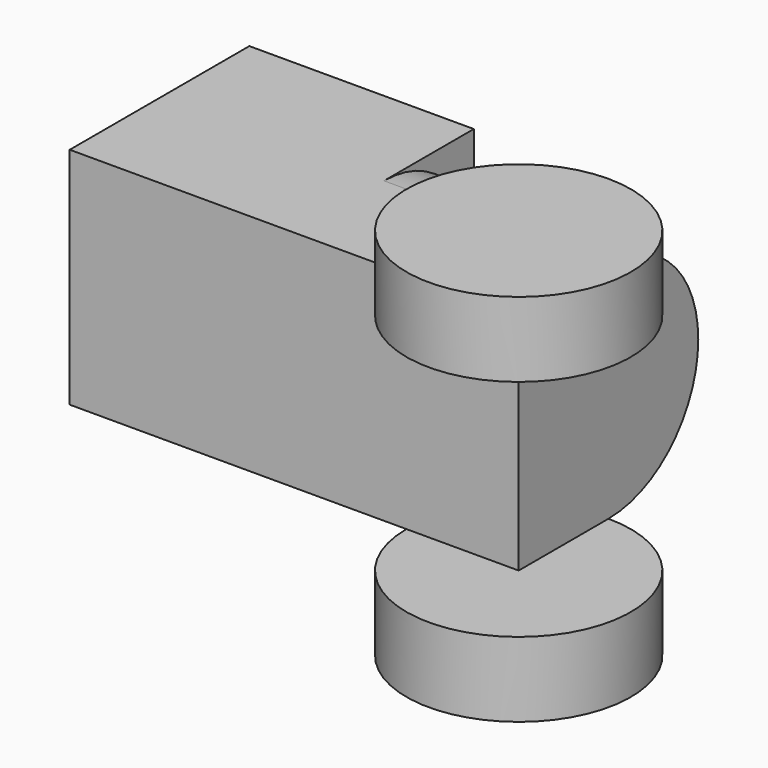
from build123d import *

# Parameters (mm, degrees)
F0_W     = 38.1
F0_H     = 38.1
F1_DEPTH = 38.1
F3_DEPTH = 38.1
F4_DEPTH = 19.05
F7_DEPTH = 12.7
F8_DEPTH = 12.7


# Not quite as in the source:
# - a feature of the source that left no trace in its solid (it failed there, or was rolled back) is left out


with BuildPart() as f1:
    # F0 (on Front) → F1 (new body)
    with BuildSketch(Plane.XZ):
        with Locations((-45.594806087, -5.8171211302)):
            Rectangle(F0_W, F0_H)
    extrude(amount=F1_DEPTH)

    # F2 (on face) → F3 (join)
    with BuildSketch(Plane.YZ.offset(-26.544806087)):
        with BuildLine():
            Line((-19.05, 13.2328788698), (-19.05, -24.8671211302))
            ThreePointArc((-19.05, -24.8671211302), (-5.5796158184, -19.2875053118), (0, -5.8171211302))
            ThreePointArc((0, -5.8171211302), (-5.5796158184, 7.6532630514), (-19.05, 13.2328788698))
        make_face()
    extrude(amount=F3_DEPTH)

    # F4 (add): a face of the model
    f4_faces = [f1.faces().sort_by_distance(p)[0] for p in [
        (-7.494806087, -19.05, -5.8171211302),
    ]]
    extrude(f4_faces, amount=F4_DEPTH)

    # F6 (on face) → F7 (join)
    with BuildSketch(Plane.XY.offset(13.2328788698)):
        with BuildLine():
            ThreePointArc((-7.494806087, -38.1), (11.555193913, -57.15), (30.605193913, -38.1))
            ThreePointArc((30.605193913, -38.1), (25.0255780946, -24.6296158184), (11.555193913, -19.05))
            Line((11.555193913, -19.05), (11.555193913, -38.1))
            Line((11.555193913, -38.1), (-7.494806087, -38.1))
        make_face()
        with BuildLine():
            Line((11.555193913, -38.1), (11.555193913, -19.05))
            ThreePointArc((11.555193913, -19.05), (-1.9151902686, -24.6296158184), (-7.494806087, -38.1))
            Line((-7.494806087, -38.1), (11.555193913, -38.1))
        make_face()
    extrude(amount=F7_DEPTH)

    # F5 (on face) → F8 (join)
    with BuildSketch(Plane(origin=(0, 0, -24.8671211302), x_dir=(1, 0, 0), z_dir=(0, 0, -1))):
        with BuildLine():
            Line((11.555193913, 38.1), (11.555193913, 19.05))
            ThreePointArc((11.555193913, 19.05), (25.0255780946, 24.6296158184), (30.605193913, 38.1))
            ThreePointArc((30.605193913, 38.1), (11.555193913, 57.15), (-7.494806087, 38.1))
            Line((-7.494806087, 38.1), (11.555193913, 38.1))
        make_face()
        with BuildLine():
            ThreePointArc((-7.494806087, 38.1), (-1.9151902686, 24.6296158184), (11.555193913, 19.05))
            Line((11.555193913, 19.05), (11.555193913, 38.1))
            Line((11.555193913, 38.1), (-7.494806087, 38.1))
        make_face()
    extrude(amount=F8_DEPTH)


solid = f1.part
